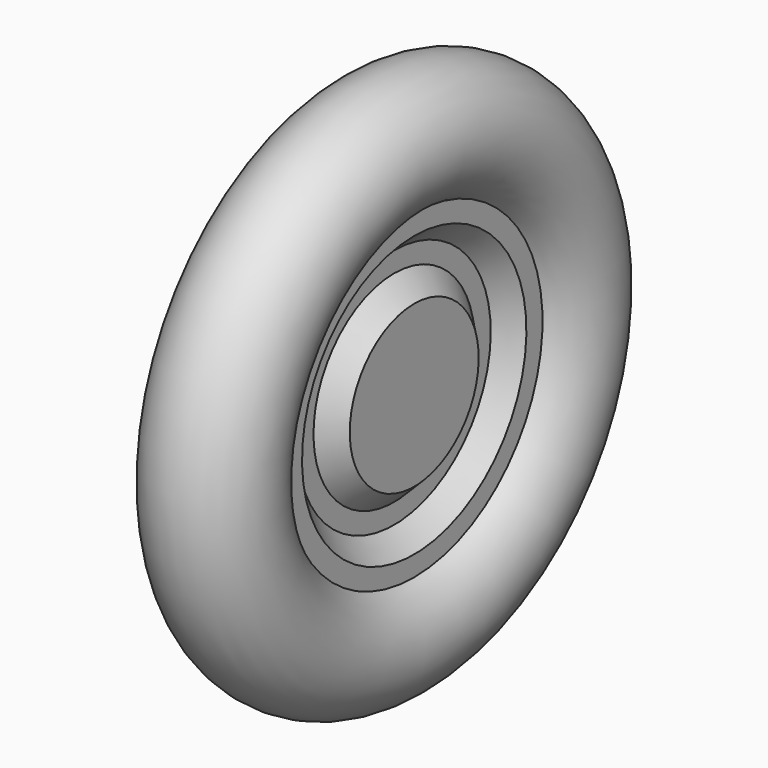
from build123d import *


# Not quite as in the source:
# - a feature names something its author has since deleted; it is built from what else it names


with BuildPart() as f1:
    # F0 (on Front) → F1 (revolve)
    with BuildSketch(Plane.XZ):
        with BuildLine():
            Line((-28.4126295149, 14.8122454338), (-28.4126295149, 19.8122454338))
            ThreePointArc((-28.4126295149, 19.8122454338), (-35.9126295149, 47.8026264906), (-43.4126295149, 19.8122454338))
            Line((-43.4126295149, 19.8122454338), (-43.4126295149, 12))
            Line((-43.4126295149, 12), (-31.4126295149, 0))
            Line((-31.4126295149, 0), (-31.4126295149, -1.8659040798))
            Line((-31.4126295149, -1.8659040798), (-31.4126295149, -20))
            Line((-31.4126295149, -20), (-28.4126295149, -20))
            Line((-28.4126295149, -20), (-28.4126295149, 0))
            Line((-28.4126295149, 0), (-33.4126295149, 5))
            Line((-33.4126295149, 5), (-33.4126295149, 10))
            Line((-33.4126295149, 10), (-28.4126295149, 14.8122454338))
        make_face()
    revolve(axis=Axis((-29.9126295149, 0, -20), (-1, 0, 0)))


solid = f1.part
